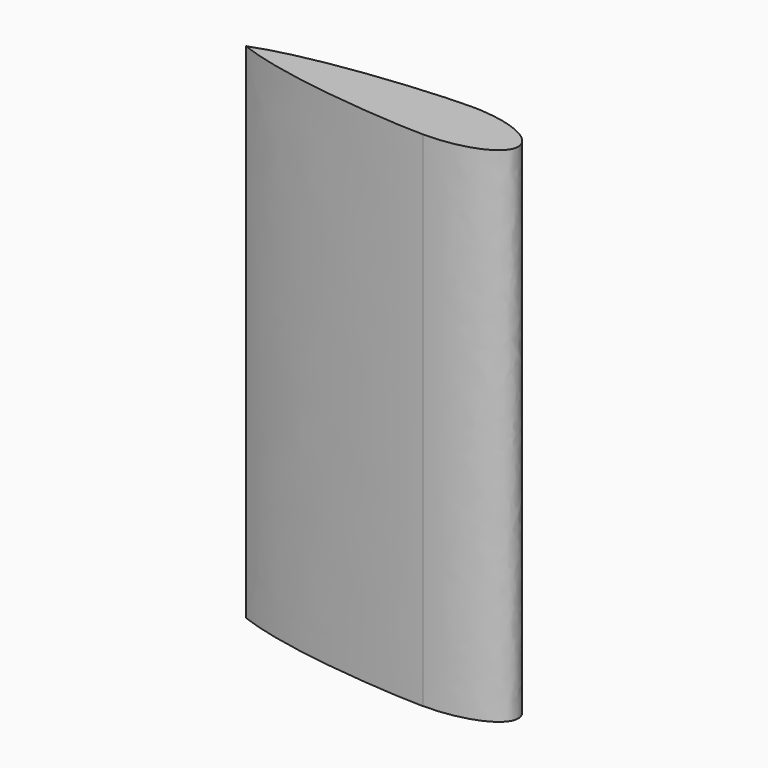
from build123d import *

# Parameters (mm, degrees)
F1_DEPTH = 250


# Not quite as in the source:
# - ends of sketch curves that miss each other by under 0.0002 mm in the source are joined


with BuildPart() as f1:
    # F0 (on Top) → F1 (new body)
    with BuildSketch(Plane.XY):
        with BuildLine():
            add(Edge.make_bspline(
                [(0, -15), (35.3319384158, -15), (35.3319384158, 0), (35.3319384158, 15), (0, 15)],
                knots=[1.5707963268, 1.5707963268, 1.5707963268, 3.1415926536, 3.1415926536, 4.7123889804, 4.7123889804, 4.7123889804], degree=2, weights=[1, 0.7071067812, 1, 0.7071067812, 1]))
            add(Edge.make_bspline(
                [(0, 15), (-16.2319140521, 15.0000000963), (-71.5773864947, 10.9885398261), (-100.0000014291, -1.909e-07)],
                knots=[0, 0, 0, 0, 101.1187435224, 101.1187435224, 101.1187435224, 101.1187435224], degree=3))
            add(Edge.make_bspline(
                [(0, -15), (-16.2319140521, -15.0000000963), (-71.5773864947, -10.9885398261), (-100.0000014291, -1.909e-07)],
                knots=[0, 0, 0, 0, 101.1187435224, 101.1187435224, 101.1187435224, 101.1187435224], degree=3))
        make_face()
    extrude(amount=-F1_DEPTH)


solid = f1.part
